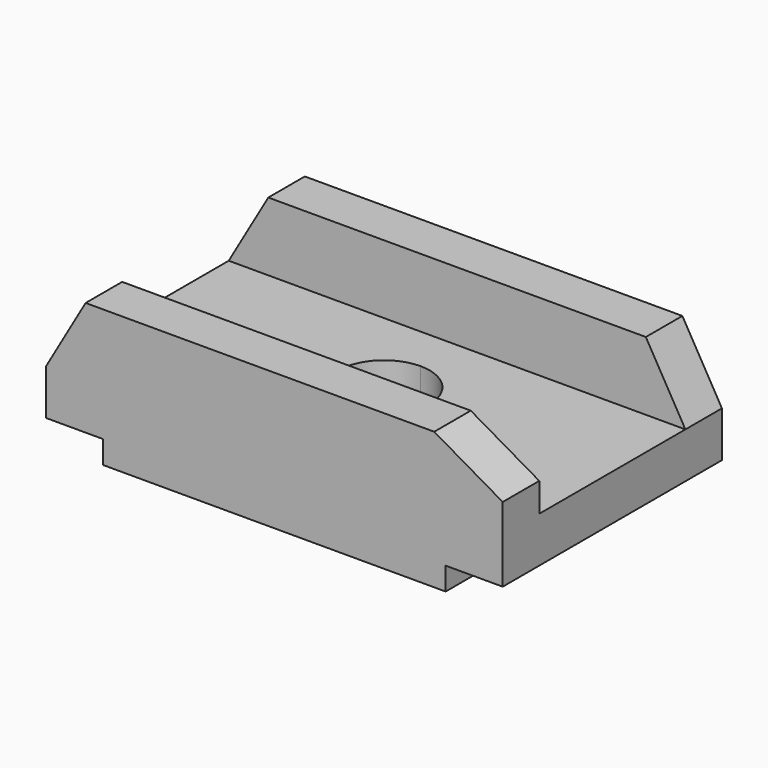
from build123d import *

# Parameters (mm, degrees)
F1_DEPTH    = 76.2
F2_W        = 127
F2_H        = 50.8
F3_DEPTH    = 19.05
F4_C1_SIZE2 = 10.9985226281
F4_C1_SIZE  = 19.05
F4_C2_SIZE2 = 10.9985226281
F4_C2_SIZE  = 19.05
F4_C3_SIZE2 = 19.05
F4_C3_SIZE  = 10.9985226281
F4_C4_SIZE2 = 19.05
F4_C4_SIZE  = 10.9985226281
F6_DEPTH    = 56.642


with BuildPart() as f1:
    # F0 (on Front) → F1 (new body)
    with BuildSketch(Plane.XZ):
        Polygon((15.875, 6.35), (15.875, 0), (111.125, 0), (111.125, 6.35), (127, 6.35), (127, 19.05), (127, 38.1), (0, 38.1), (0, 19.05), (0, 6.35), align=None)
    extrude(amount=F1_DEPTH)

    # F2 (on face) → F3 (cut)
    with BuildSketch(Plane.XY.offset(38.1)):
        with Locations((63.5, -38.1)):
            Rectangle(F2_W, F2_H)
    extrude(amount=-F3_DEPTH, mode=Mode.SUBTRACT)

    # F4: chamfer of 19.05 x 10.9985226281 on 4 edges, made by hand

    # F4_c1
    f4_c1_edges = [f1.edges().sort_by_distance(p)[0] for p in [
        (0, -69.85, 38.1),
    ]]
    f4_c1_side = f1.faces().sort_by_distance((0, -69.85, 37.8800295474))[0]
    chamfer(f4_c1_edges, length=F4_C1_SIZE, length2=F4_C1_SIZE2, reference=f4_c1_side)

    # F4_c2
    f4_c2_edges = [f1.edges().sort_by_distance(p)[0] for p in [
        (0, -6.35, 38.1),
    ]]
    f4_c2_side = f1.faces().sort_by_distance((0, -6.35, 37.8800295474))[0]
    chamfer(f4_c2_edges, length=F4_C2_SIZE, length2=F4_C2_SIZE2, reference=f4_c2_side)

    # F4_c3
    f4_c3_edges = [f1.edges().sort_by_distance(p)[0] for p in [
        (127, -6.35, 38.1),
    ]]
    f4_c3_side = f1.faces().sort_by_distance((126.7800295474, -6.35, 38.1))[0]
    chamfer(f4_c3_edges, length=F4_C3_SIZE, length2=F4_C3_SIZE2, reference=f4_c3_side)

    # F4_c4
    f4_c4_edges = [f1.edges().sort_by_distance(p)[0] for p in [
        (127, -69.85, 38.1),
    ]]
    f4_c4_side = f1.faces().sort_by_distance((127, -69.85, 37.8800295474))[0]
    chamfer(f4_c4_edges, length=F4_C4_SIZE, length2=F4_C4_SIZE2, reference=f4_c4_side)

    # F5 (on face) → F6 (cut)
    with BuildSketch(Plane.XY.offset(19.05)):
        with BuildLine():
            ThreePointArc((76.2, -38.1), (72.4802561211, -29.1197438789), (63.5, -25.4))
            ThreePointArc((63.5, -25.4), (54.5197438789, -47.0802561211), (76.2, -38.1))
        make_face()
    extrude(amount=-F6_DEPTH, mode=Mode.SUBTRACT)


solid = f1.part
